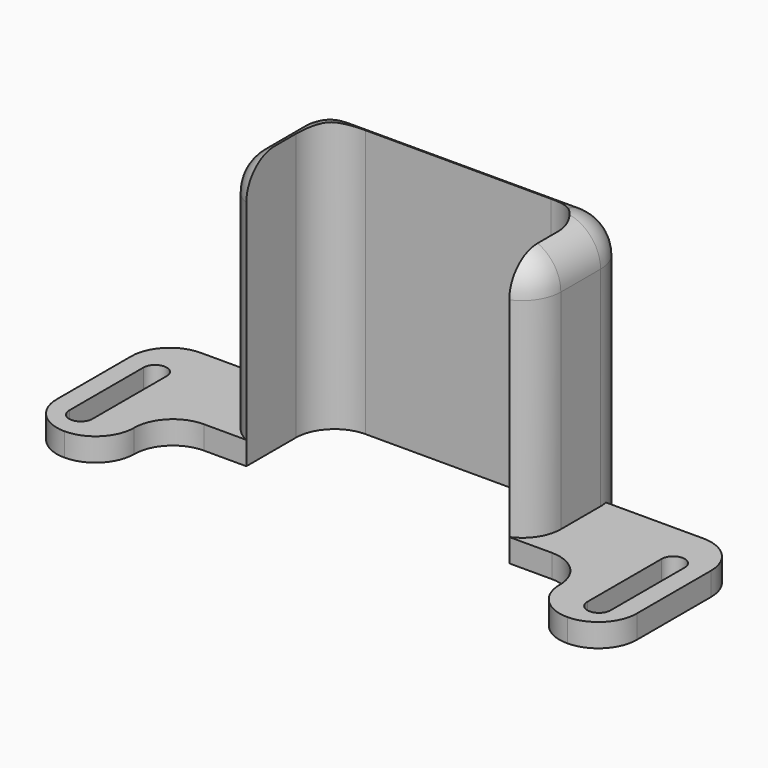
from build123d import *

# Parameters (mm, degrees)
F2_DEPTH     = 35
F3_DEPTH     = 3
F4_DEPTH     = 25
F5_R         = 4.99999
F6_T1_DEPTH  = 35
F6_T3_DEPTH  = 35
F6_T8_DEPTH  = 60
F6_T13_DEPTH = 60
F6_T15_DEPTH = 43.4564392374
F6_T20_DEPTH = 60
F6_T25_DEPTH = 60
F6_T27_DEPTH = 43.4564392374
F7_T1_DEPTH  = 6.417424305
F7_T3_DEPTH  = 30
F7_T6_ANGLE  = 89.9999999974
F7_T8_ANGLE  = 89.9999999974
F7_T10_ANGLE = 209.6926070845
F7_T12_ANGLE = 209.6926070845


# Not quite as in the source:
# - a fillet or chamfer that OpenCascade refuses, or shapes differently, is made with other operations: its cross-section is extruded or revolved along the edge and cut away or added
# - a fillet or chamfer is up to 0.001 mm smaller than in the source, because OpenCascade refuses the exact size


with BuildPart() as f2:
    # F0 (on Top) → F2 (new body)
    with BuildSketch(Plane.XY):
        Polygon((20, 26), (0, 26), (-20, 26), (-20, 22), (-20, 10), (-17, 10), (-17, 23), (0, 23), (17, 23), (17, 10), (20, 10), (20, 22), align=None)
    extrude(amount=F2_DEPTH)

    # F0 (on Top) → F3 (join)
    with BuildSketch(Plane.XY):
        Polygon((-20, 10), (-20, 22), (-37.5, 22), (-37.5, 0), (-27.5, 0), (-27.5, 10), align=None)
        Polygon((37.5, 22), (20, 22), (20, 10), (27.5, 10), (27.5, 0), (37.5, 0), align=None)
    extrude(amount=F3_DEPTH)

    # F1 (on Top) → F4 (cut)
    with BuildSketch(Plane.XY):
        with BuildLine():
            Line((35, 3.8767794613), (35, 15.8767794613))
            ThreePointArc((35, 15.8767794613), (33.5, 17.3767794613), (32, 15.8767794613))
            Line((32, 15.8767794613), (32, 3.8767794613))
            ThreePointArc((32, 3.8767794613), (33.5, 2.3767794613), (35, 3.8767794613))
        make_face()
        with BuildLine():
            ThreePointArc((-32, 15.8767794613), (-33.5, 17.3767794613), (-35, 15.8767794613))
            Line((-35, 15.8767794613), (-35, 3.8767794613))
            ThreePointArc((-35, 3.8767794613), (-33.5, 2.3767794613), (-32, 3.8767794613))
            Line((-32, 3.8767794613), (-32, 15.8767794613))
        make_face()
    extrude(amount=F4_DEPTH, mode=Mode.SUBTRACT)

    # F5 (radius 5 in the source; OpenCascade refuses exactly that, so slightly less here)
    f5_edges = [f2.edges().sort_by_distance(p)[0] for p in [
        (-37.5, 0, 1.5),
        (-27.5, 0, 1.5),
        (-37.5, 22, 1.5),
        (37.5, 22, 1.5),
        (37.5, 0, 1.5),
        (27.5, 0, 1.5),
        (27.5, 10, 1.5),
        (-27.5, 10, 1.5),
    ]]
    fillet(f5_edges, radius=F5_R)

    # F6: fillet of radius 5 on 6 edges, made by hand

    # F6_s2 → F6_t1 (join)
    with BuildSketch(Plane.XY):
        with BuildLine():
            ThreePointArc((17, 18), (15.5355339059, 21.5355339059), (12, 23))
            Line((12, 23), (17, 23))
            Line((17, 23), (17, 18))
        make_face()
    extrude(amount=F6_T1_DEPTH)

    # F6_s4 → F6_t3 (join)
    with BuildSketch(Plane.XY):
        with BuildLine():
            ThreePointArc((-12, 23), (-15.5355339059, 21.5355339059), (-17, 18))
            Line((-17, 18), (-17, 23))
            Line((-17, 23), (-12, 23))
        make_face()
    extrude(amount=F6_T3_DEPTH)


with BuildPart() as f6_tool6:
    # F6_s7 → F6_t8 (new body)
    with BuildSketch(Plane.XY.offset(-12.5)):
        with BuildLine():
            ThreePointArc((20, 21), (18.5355339059, 24.5355339059), (15, 26))
            Line((15, 26), (20, 26))
            Line((20, 26), (20, 21))
        make_face()
    extrude(amount=F6_T8_DEPTH)

    split(bisect_by=Plane.XZ.offset(-22), keep=Keep.BOTTOM)


with BuildPart() as f2_1:
    add(f2.part)

    # F6_t5: cut F6_tool6
    add(f6_tool6.part, mode=Mode.SUBTRACT)


with BuildPart() as f6_tool11:
    # F6_s12 → F6_t13 (new body)
    with BuildSketch(Plane.XY.offset(-12.5)):
        with BuildLine():
            ThreePointArc((20, 21), (18.5355339059, 24.5355339059), (15, 26))
            Line((15, 26), (20, 26))
            Line((20, 26), (20, 21))
        make_face()
    extrude(amount=F6_T13_DEPTH)

    split(bisect_by=Plane.XY.offset(3), keep=Keep.TOP)


with BuildPart() as f2_2:
    add(f2_1.part)

    # F6_t10: cut F6_tool11
    add(f6_tool11.part, mode=Mode.SUBTRACT)

    # F6_s16 → F6_t15 (cut)
    with BuildSketch(Plane.XY.offset(3)):
        with BuildLine():
            ThreePointArc((20, 14.582575695), (19.1833001327, 11.8439629074), (17, 10))
            Line((17, 10), (20, 10))
            Line((20, 10), (20, 14.582575695))
        make_face()
    extrude(amount=F6_T15_DEPTH, mode=Mode.SUBTRACT)


with BuildPart() as f6_tool18:
    # F6_s19 → F6_t20 (new body)
    with BuildSketch(Plane.XY.offset(-12.5)):
        with BuildLine():
            ThreePointArc((-20, 21), (-18.5355339059, 24.5355339059), (-15, 26))
            Line((-15, 26), (-20, 26))
            Line((-20, 26), (-20, 21))
        make_face()
    extrude(amount=F6_T20_DEPTH)

    split(bisect_by=Plane.XZ.offset(-22), keep=Keep.BOTTOM)


with BuildPart() as f2_3:
    add(f2_2.part)

    # F6_t17: cut F6_tool18
    add(f6_tool18.part, mode=Mode.SUBTRACT)


with BuildPart() as f6_tool23:
    # F6_s24 → F6_t25 (new body)
    with BuildSketch(Plane.XY.offset(-12.5)):
        with BuildLine():
            ThreePointArc((-20, 21), (-18.5355339059, 24.5355339059), (-15, 26))
            Line((-15, 26), (-20, 26))
            Line((-20, 26), (-20, 21))
        make_face()
    extrude(amount=F6_T25_DEPTH)

    split(bisect_by=Plane.XY.offset(3), keep=Keep.TOP)


with BuildPart() as f2_4:
    add(f2_3.part)

    # F6_t22: cut F6_tool23
    add(f6_tool23.part, mode=Mode.SUBTRACT)

    # F6_s28 → F6_t27 (cut)
    with BuildSketch(Plane.XY.offset(3)):
        with BuildLine():
            ThreePointArc((-20, 14.582575695), (-19.1833001327, 11.8439629074), (-17, 10))
            Line((-17, 10), (-20, 10))
            Line((-20, 10), (-20, 14.582575695))
        make_face()
    extrude(amount=F6_T27_DEPTH, mode=Mode.SUBTRACT)

    # F7: fillet of radius 5 on 3 edges, made by hand

    # F7_s2 → F7_t1 (cut)
    with BuildSketch(Plane.XZ.offset(-21)):
        with BuildLine():
            ThreePointArc((-15, 35), (-18.5355339059, 33.5355339059), (-20, 30))
            Line((-20, 30), (-20, 35))
            Line((-20, 35), (-15, 35))
        make_face()
        with BuildLine():
            ThreePointArc((15, 35), (18.5355339059, 33.5355339059), (20, 30))
            Line((20, 30), (20, 35))
            Line((20, 35), (15, 35))
        make_face()
    extrude(amount=F7_T1_DEPTH, mode=Mode.SUBTRACT)

    # F7_s4 → F7_t3 (cut)
    with BuildSketch(Plane.YZ.offset(-15)):
        with BuildLine():
            ThreePointArc((21, 35), (24.5355339059, 33.5355339059), (26, 30))
            Line((26, 30), (26, 35))
            Line((26, 35), (21, 35))
        make_face()
    extrude(amount=F7_T3_DEPTH, mode=Mode.SUBTRACT)

    # F7_s5 → F7_t6 (revolve, cut)
    with BuildSketch(Plane.YZ.offset(14.9999999999)):
        with BuildLine():
            ThreePointArc((21, 35), (24.5355339059, 33.5355339059), (26, 30))
            Line((26, 30), (26, 35))
            Line((26, 35), (21, 35))
        make_face()
    revolve(axis=Axis((14.9999999999, 20.9999999999, 35), (0, 0, -1)), revolution_arc=F7_T6_ANGLE, mode=Mode.SUBTRACT)

    # F7_s7 → F7_t8 (revolve, cut)
    with BuildSketch(Plane.XZ.offset(-20.9999999999)):
        with BuildLine():
            ThreePointArc((-15, 35), (-18.5355339059, 33.5355339059), (-20, 30))
            Line((-20, 30), (-20, 35))
            Line((-20, 35), (-15, 35))
        make_face()
    revolve(axis=Axis((-14.9999999999, 20.9999999999, 35), (0, 0, -1)), revolution_arc=F7_T8_ANGLE, mode=Mode.SUBTRACT)

    # F7_s9 → F7_t10 (revolve, cut)
    with BuildSketch(Plane.XZ.offset(-14.5825756948)):
        with BuildLine():
            ThreePointArc((20, 30), (18.5355339059, 33.5355339059), (15, 35))
            Line((15, 35), (20, 35))
            Line((20, 35), (20, 30))
        make_face()
    revolve(axis=Axis((15.0000000002, 14.5825756948, 35), (0, 0, -1)), revolution_arc=F7_T10_ANGLE, mode=Mode.SUBTRACT)

    # F7_s11 → F7_t12 (revolve, cut)
    with BuildSketch(Plane(origin=(-9.9554834358, 17.4590545428, 0), x_dir=(0, 0, 1), z_dir=(-0.4953465841, 0.8686954366, 0))):
        with BuildLine():
            ThreePointArc((35, -5.8070024913), (33.5355339059, -2.2714685854), (30, -0.8070024913))
            Line((30, -0.8070024913), (35, -0.8070024913))
            Line((35, -0.8070024913), (35, -5.8070024913))
        make_face()
    revolve(axis=Axis((-15.0000000002, 14.5825756948, 35), (0, 0, -1)), revolution_arc=F7_T12_ANGLE, mode=Mode.SUBTRACT)


solid = f2_4.part
